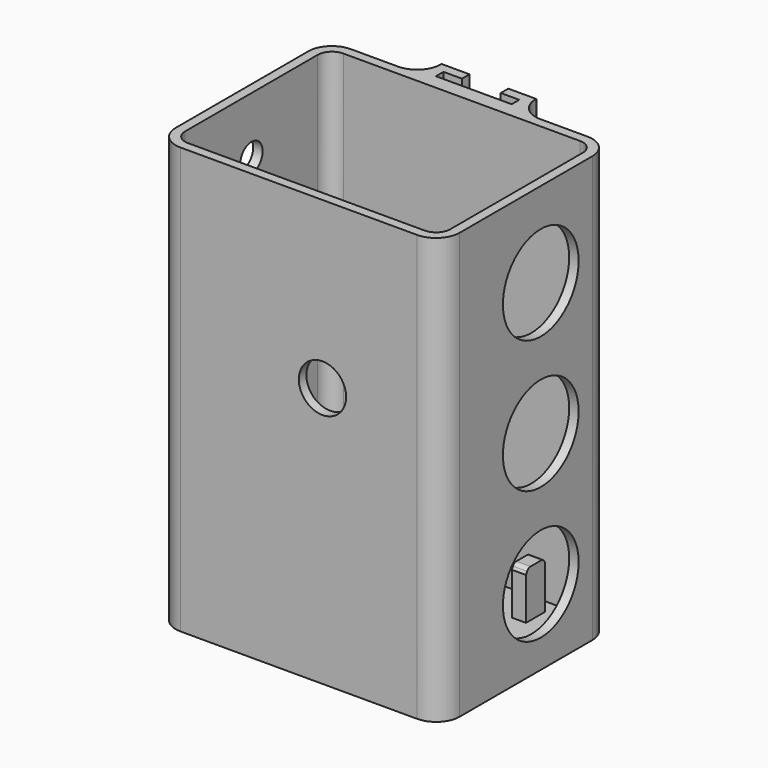
from build123d import *

# Parameters (mm, degrees)
F1_DEPTH  = 90
F2_T      = -2
F4_DEPTH  = 90
F5_R      = 5
F6_DEPTH  = 25
F7_W      = 10.9698139131
F7_H      = 3
F7_W_2    = 3
F7_H_2    = 5
F8_DEPTH  = 10
F10_DEPTH = 70
F11_R     = 10
F12_DEPTH = 20
F13_R     = 5
F14_SIZE2 = 5
F14_SIZE  = 2
F15_R     = 1
F16_R     = 2.95
F17_DEPTH = 25


# Not quite as in the source:
# - a feature names something its author has since deleted; it is built from what else it names


with BuildPart() as f1:
    # F0 (on Top) → F1 (new body)
    with BuildSketch(Plane.XY):
        with BuildLine():
            Line((-35, -116), (0, -116))
            Line((0, -116), (15, -116))
            ThreePointArc((15, -116), (18.5355339059, -114.5355339059), (20, -111))
            Line((20, -111), (20, -76))
            ThreePointArc((20, -76), (18.5355339059, -72.4644660941), (15, -71))
            Line((15, -71), (-35, -71))
            ThreePointArc((-35, -71), (-38.5355339059, -72.4644660941), (-40, -76))
            Line((-40, -76), (-40, -111))
            ThreePointArc((-40, -111), (-38.5355339059, -114.5355339059), (-35, -116))
        make_face()
    extrude(amount=F1_DEPTH)

    # F2
    f2_openings = [f1.faces().sort_by_distance(p)[0] for p in [
        (-10, -93.5, 90),
    ]]
    offset(amount=F2_T, openings=f2_openings)

    # F3 (on face) → F4 (join, through all)
    with BuildSketch(Plane.XY.offset(90)):
        Polygon((-20, -65.7917543815), (-20, -71), (-10, -71), (0, -71), (0, -65.7917543815), (-5.9066830128, -65.7917543815), (-5.9066830128, -67.7917543815), (-2, -67.7917543815), (-2, -69.7917543815), (-18, -69.7917543815), (-18, -67.7917543815), (-14.0933169872, -67.7917543815), (-14.0933169872, -65.7917543815), align=None)
    extrude(amount=-F4_DEPTH)

    # F5 (on face) → F6 (cut)
    with BuildSketch(Plane.XZ.offset(116)):
        with Locations((-5, 55)):
            Circle(F5_R)
    extrude(amount=-F6_DEPTH, mode=Mode.SUBTRACT)

    # F7 (on face) → F8 (join)
    with BuildSketch(Plane.XY.offset(2)):
        with Locations((-16.3644514978, -74.5)):
            Rectangle(F7_W, F7_H)
        with Locations((8.5, -78.5)):
            Rectangle(F7_W_2, F7_H_2)
        with Locations((8.5, -98.5)):
            Rectangle(F7_W_2, F7_H_2)
    extrude(amount=F8_DEPTH)

    # F9 (on face) → F10 (join)
    with BuildSketch(Plane.XY.offset(2)):
        Polygon((-34, -101), (-38, -101), (-38, -107), (-34, -107), (-34, -105), (-36, -105), (-36, -103), (-34, -103), align=None)
        Polygon((7, -101), (2, -101), (2, -103), (4, -103), (4, -105), (2, -105), (2, -107), (7, -107), (7, -114), (10, -114), (10, -107), (10, -101), align=None)
    extrude(amount=F10_DEPTH)

    # F11 (on face) → F12 (cut)
    with BuildSketch(Plane.YZ.offset(20)):
        with Locations((-89.6050930023, 72)):
            Circle(F11_R)
        with Locations((-89.6050930023, 44)):
            Circle(F11_R)
        with Locations((-89.6050930023, 16)):
            Circle(F11_R)
    extrude(amount=-F12_DEPTH, mode=Mode.SUBTRACT)

    # F13
    f13_edges = [f1.edges().sort_by_distance(p)[0] for p in [
        (0, -71, 45),
        (-20, -71, 45),
    ]]
    fillet(f13_edges, radius=F13_R)

    # F14
    f14_edges = [f1.edges().sort_by_distance(p)[0] for p in [
        (-16.364451, -76, 12),
    ]]
    f14_side = f1.faces().sort_by_distance((-16.364451, -74.5, 12))[0]
    chamfer(f14_edges, length=F14_SIZE, length2=F14_SIZE2, reference=f14_side)

    # F15
    f15_edges = [f1.edges().sort_by_distance(p)[0] for p in [
        (8.5, -80.439942, 12),
        (8.5, -76, 12),
        (8.5, -98.770244, 12),
        (8.5, -96, 8.312012),
    ]]
    fillet(f15_edges, radius=F15_R)

    # F16 (on face) → F17 (cut)
    with BuildSketch(Plane(origin=(-40, 0, 0), x_dir=(0, -1, 0), z_dir=(-1, 0, 0))):
        with Locations((93.5, 78)):
            Circle(F16_R)
    extrude(amount=-F17_DEPTH, mode=Mode.SUBTRACT)


solid = f1.part
